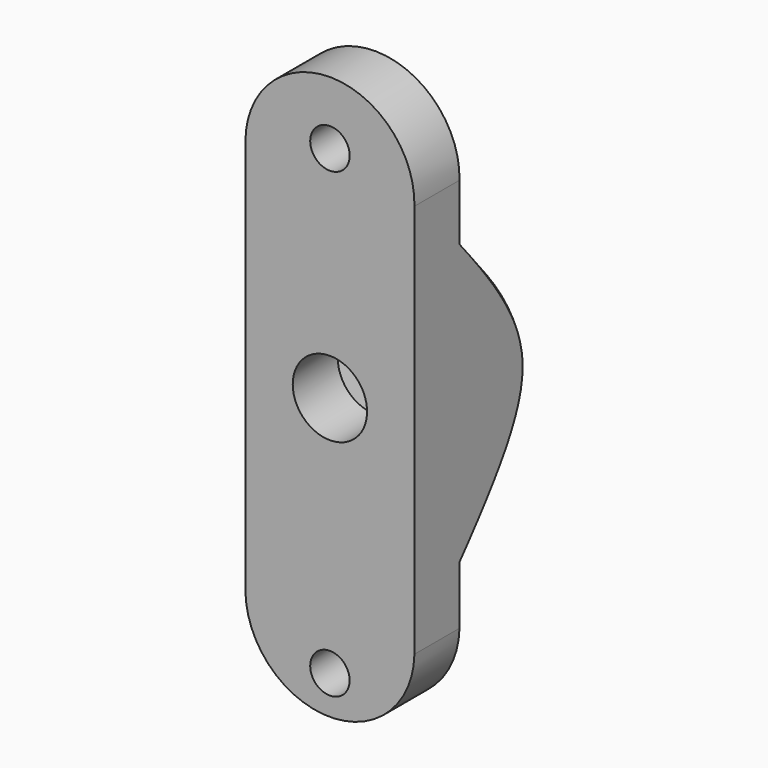
from build123d import *

# Parameters (mm, degrees)
F1_DEPTH     = 5
F2_R         = 7.5
F3_DEPTH     = 7
F5_D         = 6.6
F7_DEPTH     = 7
F9_T4_ANGLE  = 179.9999997857
F9_T10_ANGLE = 180.0000002143
F10_D        = 3.5


# Not quite as in the source:
# - a fillet or chamfer that OpenCascade refuses, or shapes differently, is made with other operations: its cross-section is extruded or revolved along the edge and cut away or added


with BuildPart() as f1:
    # F0 (on Front) → F1 (new body)
    with BuildSketch(Plane.XZ):
        with BuildLine():
            ThreePointArc((-7.5, -17.4188318139), (-0.0794529453, -24.9192617628), (7.5, -17.5794483415))
            Line((7.5, -17.5794483415), (7.5, 17.4188318139))
            ThreePointArc((7.5, 17.4188318139), (0.0811727899, 25.0798782903), (-7.5, 17.5794483415))
            Line((-7.5, 17.5794483415), (-7.5, -17.4188318139))
        make_face()
    extrude(amount=F1_DEPTH)

    # F2 (on face) → F3 (join)
    with BuildSketch(Plane(origin=(0, 0, 0), x_dir=(-1, 0, 0), z_dir=(0, 1, 0))):
        Circle(F2_R)
    extrude(amount=F3_DEPTH)

    # F5 (through all)
    with Locations(Plane.XZ.offset(5)):
        with Locations((0, 0)):
            Hole(F5_D / 2)

    # F6 (on face) → F7 (cut, through all)
    with BuildSketch(Plane(origin=(0, 7, 0), x_dir=(-1, 0, 0), z_dir=(0, 1, 0))):
        Polygon((2.9589201296, -5.125), (5.9178402592, 0), (2.9589201296, 5.125), (-2.9589201296, 5.125), (-5.9178402592, 0), (-2.9589201296, -5.125), align=None)
    extrude(amount=-F7_DEPTH, mode=Mode.SUBTRACT)

    # F9: chamfer of 7 on 2 edges, made by hand


with BuildPart() as f9_tool2:
    # F9_s3 → F9_t4 (revolve)
    with BuildSketch(Plane.XY):
        Polygon((-14.5, 0), (-7.5, 7), (-7.5, 0), align=None)
    revolve(axis=Axis((0, 0, 0), (0, 1, 0)), revolution_arc=F9_T4_ANGLE)

    split(bisect_by=Plane.YZ.offset(-7.5), keep=Keep.TOP)

    split(bisect_by=Plane.YZ.offset(7.5), keep=Keep.BOTTOM)


with BuildPart() as f1_1:
    add(f1.part)

    # F9_t1: union F9_tool2
    add(f9_tool2.part)


with BuildPart() as f9_tool8:
    # F9_s9 → F9_t10 (revolve)
    with BuildSketch(Plane.XY):
        Polygon((14.5, 0), (7.5, 7), (7.5, 0), align=None)
    revolve(axis=Axis((0, 0, 0), (0, 1, 0)), revolution_arc=F9_T10_ANGLE)

    split(bisect_by=Plane.YZ.offset(-7.5), keep=Keep.TOP)

    split(bisect_by=Plane.YZ.offset(7.5), keep=Keep.BOTTOM)


with BuildPart() as f1_2:
    add(f1_1.part)

    # F9_t7: union F9_tool8
    add(f9_tool8.part)

    # F10 (through all)
    with Locations(Plane.XZ.offset(5)):
        with Locations((0.0010000484, 19.5), (0, -21.5)):
            Hole(F10_D / 2)


solid = f1_2.part
